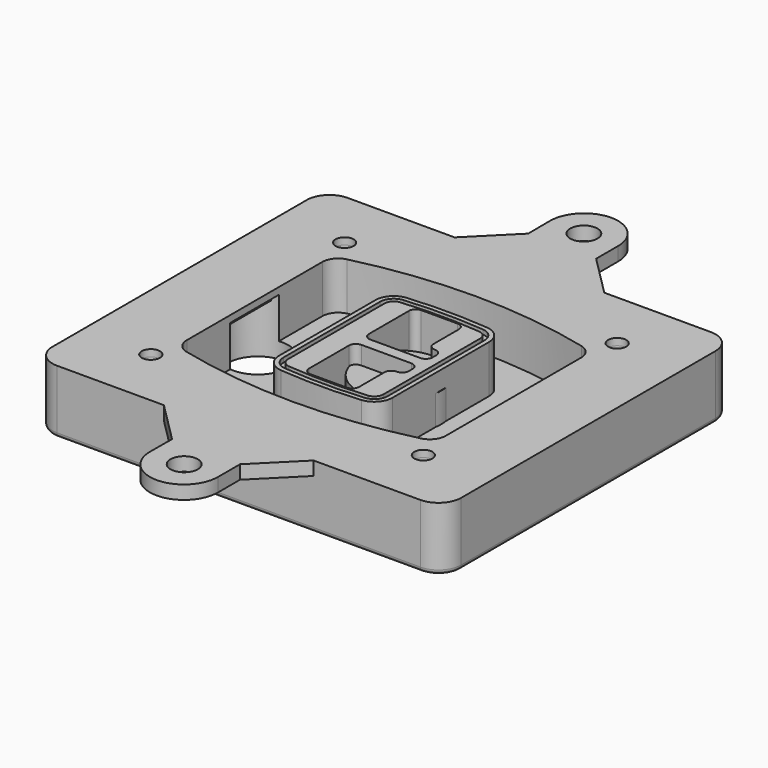
from build123d import *

# Parameters (mm, degrees)
F0_R      = 4
F1_DEPTH  = 25
F2_DEPTH  = 3
F3_DEPTH  = 18
F5_DEPTH  = 21
F6_DEPTH  = 2
F8_DEPTH  = 20
F9_DEPTH  = 16
F10_DEPTH = 25
F7_R      = 6
F7_R_2    = 4
F11_DEPTH = 6
F13_DEPTH = 9
F15_R     = 2
F16_R     = 4
F16_R_2   = 6
F17_DEPTH = 3


# Not quite as in the source:
# - a feature of the source that left no trace in its solid (it failed there, or was rolled back) is left out
# - a feature names something its author has since deleted; it is built from what else it names


with BuildPart() as f1:
    # F0 (on Top) → F1 (new body)
    with BuildSketch(Plane.XY):
        with BuildLine():
            ThreePointArc((-90, -70), (-87.0710678119, -77.0710678119), (-80, -80))
            Line((-80, -80), (80, -80))
            ThreePointArc((80, -80), (87.0710678119, -77.0710678119), (90, -70))
            Line((90, -70), (90, 70))
            ThreePointArc((90, 70), (87.0710678119, 77.0710678119), (80, 80))
            Line((80, 80), (-80, 80))
            ThreePointArc((-80, 80), (-87.0710678119, 77.0710678119), (-90, 70))
            Line((-90, 70), (-90, -70))
        make_face()
        with Locations((-60, -53.3333333333)):
            Circle(F0_R, mode=Mode.SUBTRACT)
        with Locations((60, -53.3333333333)):
            Circle(F0_R, mode=Mode.SUBTRACT)
        with BuildLine():
            ThreePointArc((-64, 37.2990447398), (-61.0143011354, 45.9411029726), (-53.3306899286, 50.8970778549))
            ThreePointArc((-53.3306899286, 50.8970778549), (0, 57.3333333333), (53.3306899286, 50.8970778549))
            ThreePointArc((53.3306899286, 50.8970778549), (61.0143011354, 45.9411029726), (64, 37.2990447398))
            Line((64, 37.2990447398), (64, -37.2990447398))
            ThreePointArc((64, -37.2990447398), (61.0143011354, -45.9411029726), (53.3306899286, -50.8970778549))
            ThreePointArc((53.3306899286, -50.8970778549), (0, -57.3333333333), (-53.3306899286, -50.8970778549))
            ThreePointArc((-53.3306899286, -50.8970778549), (-61.0143011354, -45.9411029726), (-64, -37.2990447398))
            Line((-64, -37.2990447398), (-64, 37.2990447398))
        make_face(mode=Mode.SUBTRACT)
        with Locations((-60, 53.3333333333)):
            Circle(F0_R, mode=Mode.SUBTRACT)
        with Locations((60, 53.3333333333)):
            Circle(F0_R, mode=Mode.SUBTRACT)
        with BuildLine():
            ThreePointArc((53.3306899286, 50.8970778549), (0, 57.3333333333), (-53.3306899286, 50.8970778549))
            ThreePointArc((-53.3306899286, 50.8970778549), (-61.0143011354, 45.9411029726), (-64, 37.2990447398))
            Line((-64, 37.2990447398), (-64, -37.2990447398))
            ThreePointArc((-64, -37.2990447398), (-61.0143011354, -45.9411029726), (-53.3306899286, -50.8970778549))
            ThreePointArc((-53.3306899286, -50.8970778549), (0, -57.3333333333), (53.3306899286, -50.8970778549))
            ThreePointArc((53.3306899286, -50.8970778549), (61.0143011354, -45.9411029726), (64, -37.2990447398))
            Line((64, -37.2990447398), (64, 37.2990447398))
            ThreePointArc((64, 37.2990447398), (61.0143011354, 45.9411029726), (53.3306899286, 50.8970778549))
        make_face()
        with BuildLine():
            Line((-60, -37.2990447398), (-60, 37.2990447398))
            ThreePointArc((-60, 37.2990447398), (-57.8673579538, 43.4719434775), (-52.3790642347, 47.0119255363))
            ThreePointArc((-52.3790642347, 47.0119255363), (0, 53.3333333333), (52.3790642347, 47.0119255363))
            ThreePointArc((52.3790642347, 47.0119255363), (57.8673579538, 43.4719434775), (60, 37.2990447398))
            Line((60, 37.2990447398), (60, -37.2990447398))
            ThreePointArc((60, -37.2990447398), (57.8673579538, -43.4719434775), (52.3790642347, -47.0119255363))
            ThreePointArc((52.3790642347, -47.0119255363), (0, -53.3333333333), (-52.3790642347, -47.0119255363))
            ThreePointArc((-52.3790642347, -47.0119255363), (-57.8673579538, -43.4719434775), (-60, -37.2990447398))
        make_face(mode=Mode.SUBTRACT)
        with BuildLine():
            ThreePointArc((-52.3790642347, 47.0119255363), (-57.8673579538, 43.4719434775), (-60, 37.2990447398))
            Line((-60, 37.2990447398), (-60, -37.2990447398))
            ThreePointArc((-60, -37.2990447398), (-57.8673579538, -43.4719434775), (-52.3790642347, -47.0119255363))
            ThreePointArc((-52.3790642347, -47.0119255363), (0, -53.3333333333), (52.3790642347, -47.0119255363))
            ThreePointArc((52.3790642347, -47.0119255363), (57.8673579538, -43.4719434775), (60, -37.2990447398))
            Line((60, -37.2990447398), (60, 37.2990447398))
            ThreePointArc((60, 37.2990447398), (57.8673579538, 43.4719434775), (52.3790642347, 47.0119255363))
            ThreePointArc((52.3790642347, 47.0119255363), (0, 53.3333333333), (-52.3790642347, 47.0119255363))
        make_face()
        with BuildLine():
            ThreePointArc((51.6653449643, 44.0980612973), (55.5071505677, 41.6200738562), (57, 37.2990447398))
            Line((57, 37.2990447398), (57, -37.2990447398))
            ThreePointArc((57, -37.2990447398), (55.5071505677, -41.6200738562), (51.6653449643, -44.0980612973))
            ThreePointArc((51.6653449643, -44.0980612973), (0, -50.3333333333), (-51.6653449643, -44.0980612973))
            ThreePointArc((-51.6653449643, -44.0980612973), (-55.5071505677, -41.6200738562), (-57, -37.2990447398))
            Line((-57, -37.2990447398), (-57, 37.2990447398))
            ThreePointArc((-57, 37.2990447398), (-55.5071505677, 41.6200738562), (-51.6653449643, 44.0980612973))
            ThreePointArc((-51.6653449643, 44.0980612973), (0, 50.3333333333), (51.6653449643, 44.0980612973))
        make_face(mode=Mode.SUBTRACT)
        with BuildLine():
            Line((57, -37.2990447398), (57, 37.2990447398))
            ThreePointArc((57, 37.2990447398), (55.5071505677, 41.6200738562), (51.6653449643, 44.0980612973))
            ThreePointArc((51.6653449643, 44.0980612973), (0, 50.3333333333), (-51.6653449643, 44.0980612973))
            ThreePointArc((-51.6653449643, 44.0980612973), (-55.5071505677, 41.6200738562), (-57, 37.2990447398))
            Line((-57, 37.2990447398), (-57, -37.2990447398))
            ThreePointArc((-57, -37.2990447398), (-55.5071505677, -41.6200738562), (-51.6653449643, -44.0980612973))
            ThreePointArc((-51.6653449643, -44.0980612973), (0, -50.3333333333), (51.6653449643, -44.0980612973))
            ThreePointArc((51.6653449643, -44.0980612973), (55.5071505677, -41.6200738562), (57, -37.2990447398))
        make_face()
    extrude(amount=-F1_DEPTH)

    # F0 (on Top) → F2 (join)
    with BuildSketch(Plane.XY):
        with BuildLine():
            ThreePointArc((-52.3790642347, 47.0119255363), (-57.8673579538, 43.4719434775), (-60, 37.2990447398))
            Line((-60, 37.2990447398), (-60, -37.2990447398))
            ThreePointArc((-60, -37.2990447398), (-57.8673579538, -43.4719434775), (-52.3790642347, -47.0119255363))
            ThreePointArc((-52.3790642347, -47.0119255363), (0, -53.3333333333), (52.3790642347, -47.0119255363))
            ThreePointArc((52.3790642347, -47.0119255363), (57.8673579538, -43.4719434775), (60, -37.2990447398))
            Line((60, -37.2990447398), (60, 37.2990447398))
            ThreePointArc((60, 37.2990447398), (57.8673579538, 43.4719434775), (52.3790642347, 47.0119255363))
            ThreePointArc((52.3790642347, 47.0119255363), (0, 53.3333333333), (-52.3790642347, 47.0119255363))
        make_face()
        with BuildLine():
            ThreePointArc((51.6653449643, 44.0980612973), (55.5071505677, 41.6200738562), (57, 37.2990447398))
            Line((57, 37.2990447398), (57, -37.2990447398))
            ThreePointArc((57, -37.2990447398), (55.5071505677, -41.6200738562), (51.6653449643, -44.0980612973))
            ThreePointArc((51.6653449643, -44.0980612973), (0, -50.3333333333), (-51.6653449643, -44.0980612973))
            ThreePointArc((-51.6653449643, -44.0980612973), (-55.5071505677, -41.6200738562), (-57, -37.2990447398))
            Line((-57, -37.2990447398), (-57, 37.2990447398))
            ThreePointArc((-57, 37.2990447398), (-55.5071505677, 41.6200738562), (-51.6653449643, 44.0980612973))
            ThreePointArc((-51.6653449643, 44.0980612973), (0, 50.3333333333), (51.6653449643, 44.0980612973))
        make_face(mode=Mode.SUBTRACT)
    extrude(amount=F2_DEPTH)

    # F0 (on Top) → F3 (cut)
    with BuildSketch(Plane.XY):
        with BuildLine():
            Line((57, -37.2990447398), (57, 37.2990447398))
            ThreePointArc((57, 37.2990447398), (55.5071505677, 41.6200738562), (51.6653449643, 44.0980612973))
            ThreePointArc((51.6653449643, 44.0980612973), (0, 50.3333333333), (-51.6653449643, 44.0980612973))
            ThreePointArc((-51.6653449643, 44.0980612973), (-55.5071505677, 41.6200738562), (-57, 37.2990447398))
            Line((-57, 37.2990447398), (-57, -37.2990447398))
            ThreePointArc((-57, -37.2990447398), (-55.5071505677, -41.6200738562), (-51.6653449643, -44.0980612973))
            ThreePointArc((-51.6653449643, -44.0980612973), (0, -50.3333333333), (51.6653449643, -44.0980612973))
            ThreePointArc((51.6653449643, -44.0980612973), (55.5071505677, -41.6200738562), (57, -37.2990447398))
        make_face()
    extrude(amount=-F3_DEPTH, mode=Mode.SUBTRACT)

    # F4 (on face) → F5 (join, through all)
    with BuildSketch(Plane.XY.offset(3)):
        with BuildLine():
            ThreePointArc((-25, -26.587695628), (-22.8992979869, -31.9912392117), (-17.7004291845, -34.5569740744))
            ThreePointArc((-17.7004291845, -34.5569740744), (0, -35.3333333333), (17.7004291845, -34.5569740744))
            ThreePointArc((17.7004291845, -34.5569740744), (22.8992979869, -31.9912392117), (25, -26.587695628))
            Line((25, -26.587695628), (25, 26.587695628))
            ThreePointArc((25, 26.587695628), (22.8992979869, 31.9912392117), (17.7004291845, 34.5569740744))
            ThreePointArc((17.7004291845, 34.5569740744), (0, 35.3333333333), (-17.7004291845, 34.5569740744))
            ThreePointArc((-17.7004291845, 34.5569740744), (-22.8992979869, 31.9912392117), (-25, 26.587695628))
            Line((-25, 26.587695628), (-25, -26.587695628))
        make_face()
        with BuildLine():
            ThreePointArc((17.5253218884, 32.5646544628), (21.4244734902, 30.6403533158), (23, 26.587695628))
            Line((23, 26.587695628), (23, -26.587695628))
            ThreePointArc((23, -26.587695628), (21.4244734902, -30.6403533158), (17.5253218884, -32.5646544628))
            ThreePointArc((17.5253218884, -32.5646544628), (0, -33.3333333333), (-17.5253218884, -32.5646544628))
            ThreePointArc((-17.5253218884, -32.5646544628), (-21.4244734902, -30.6403533158), (-23, -26.587695628))
            Line((-23, -26.587695628), (-23, 26.587695628))
            ThreePointArc((-23, 26.587695628), (-21.4244734902, 30.6403533158), (-17.5253218884, 32.5646544628))
            ThreePointArc((-17.5253218884, 32.5646544628), (0, 33.3333333333), (17.5253218884, 32.5646544628))
        make_face(mode=Mode.SUBTRACT)
        with BuildLine():
            Line((23, -26.587695628), (23, 26.587695628))
            ThreePointArc((23, 26.587695628), (21.4244734902, 30.6403533158), (17.5253218884, 32.5646544628))
            ThreePointArc((17.5253218884, 32.5646544628), (0, 33.3333333333), (-17.5253218884, 32.5646544628))
            ThreePointArc((-17.5253218884, 32.5646544628), (-21.4244734902, 30.6403533158), (-23, 26.587695628))
            Line((-23, 26.587695628), (-23, -26.587695628))
            ThreePointArc((-23, -26.587695628), (-21.4244734902, -30.6403533158), (-17.5253218884, -32.5646544628))
            ThreePointArc((-17.5253218884, -32.5646544628), (0, -33.3333333333), (17.5253218884, -32.5646544628))
            ThreePointArc((17.5253218884, -32.5646544628), (21.4244734902, -30.6403533158), (23, -26.587695628))
        make_face()
        with BuildLine():
            ThreePointArc((17.3502145923, 30.5723348512), (19.9496489934, 29.2894674198), (21, 26.587695628))
            Line((21, 26.587695628), (21, -26.587695628))
            ThreePointArc((21, -26.587695628), (19.9496489934, -29.2894674198), (17.3502145923, -30.5723348512))
            ThreePointArc((17.3502145923, -30.5723348512), (0, -31.3333333333), (-17.3502145923, -30.5723348512))
            ThreePointArc((-17.3502145923, -30.5723348512), (-19.9496489934, -29.2894674198), (-21, -26.587695628))
            Line((-21, -26.587695628), (-21, 26.587695628))
            ThreePointArc((-21, 26.587695628), (-19.9496489934, 29.2894674198), (-17.3502145923, 30.5723348512))
            ThreePointArc((-17.3502145923, 30.5723348512), (0, 31.3333333333), (17.3502145923, 30.5723348512))
        make_face(mode=Mode.SUBTRACT)
        with BuildLine():
            Line((21, -26.587695628), (21, 26.587695628))
            ThreePointArc((21, 26.587695628), (19.9496489934, 29.2894674198), (17.3502145923, 30.5723348512))
            ThreePointArc((17.3502145923, 30.5723348512), (0, 31.3333333333), (-17.3502145923, 30.5723348512))
            ThreePointArc((-17.3502145923, 30.5723348512), (-19.9496489934, 29.2894674198), (-21, 26.587695628))
            Line((-21, 26.587695628), (-21, -26.587695628))
            ThreePointArc((-21, -26.587695628), (-19.9496489934, -29.2894674198), (-17.3502145923, -30.5723348512))
            ThreePointArc((-17.3502145923, -30.5723348512), (0, -31.3333333333), (17.3502145923, -30.5723348512))
            ThreePointArc((17.3502145923, -30.5723348512), (19.9496489934, -29.2894674198), (21, -26.587695628))
        make_face()
        with BuildLine():
            Line((-8, -2.5), (14, -2.5))
            ThreePointArc((14, -2.5), (16.1213203436, -3.3786796564), (17, -5.5))
            Line((17, -5.5), (17, -7.5))
            ThreePointArc((17, -7.5), (16.1213203436, -9.6213203436), (14, -10.5))
            ThreePointArc((14, -10.5), (11.8786796564, -11.3786796564), (11, -13.5))
            Line((11, -13.5), (11, -27.5))
            ThreePointArc((11, -27.5), (10.1213203436, -29.6213203436), (8, -30.5))
            Line((8, -30.5), (-8, -30.5))
            ThreePointArc((-8, -30.5), (-10.1213203436, -29.6213203436), (-11, -27.5))
            Line((-11, -27.5), (-11, -5.5))
            ThreePointArc((-11, -5.5), (-10.1213203436, -3.3786796564), (-8, -2.5))
        make_face(mode=Mode.SUBTRACT)
        with BuildLine():
            ThreePointArc((-8, 2.5), (-10.1213203436, 3.3786796564), (-11, 5.5))
            Line((-11, 5.5), (-11, 27.5))
            ThreePointArc((-11, 27.5), (-10.1213203436, 29.6213203436), (-8, 30.5))
            Line((-8, 30.5), (8, 30.5))
            ThreePointArc((8, 30.5), (10.1213203436, 29.6213203436), (11, 27.5))
            Line((11, 27.5), (11, 13.5))
            ThreePointArc((11, 13.5), (11.8786796564, 11.3786796564), (14, 10.5))
            ThreePointArc((14, 10.5), (16.1213203436, 9.6213203436), (17, 7.5))
            Line((17, 7.5), (17, 5.5))
            ThreePointArc((17, 5.5), (16.1213203436, 3.3786796564), (14, 2.5))
            Line((14, 2.5), (-8, 2.5))
        make_face(mode=Mode.SUBTRACT)
    extrude(amount=-F5_DEPTH)

    # F4 (on face) → F6 (cut)
    with BuildSketch(Plane.XY.offset(3)):
        with BuildLine():
            Line((23, -26.587695628), (23, 26.587695628))
            ThreePointArc((23, 26.587695628), (21.4244734902, 30.6403533158), (17.5253218884, 32.5646544628))
            ThreePointArc((17.5253218884, 32.5646544628), (0, 33.3333333333), (-17.5253218884, 32.5646544628))
            ThreePointArc((-17.5253218884, 32.5646544628), (-21.4244734902, 30.6403533158), (-23, 26.587695628))
            Line((-23, 26.587695628), (-23, -26.587695628))
            ThreePointArc((-23, -26.587695628), (-21.4244734902, -30.6403533158), (-17.5253218884, -32.5646544628))
            ThreePointArc((-17.5253218884, -32.5646544628), (0, -33.3333333333), (17.5253218884, -32.5646544628))
            ThreePointArc((17.5253218884, -32.5646544628), (21.4244734902, -30.6403533158), (23, -26.587695628))
        make_face()
        with BuildLine():
            ThreePointArc((17.3502145923, 30.5723348512), (19.9496489934, 29.2894674198), (21, 26.587695628))
            Line((21, 26.587695628), (21, -26.587695628))
            ThreePointArc((21, -26.587695628), (19.9496489934, -29.2894674198), (17.3502145923, -30.5723348512))
            ThreePointArc((17.3502145923, -30.5723348512), (0, -31.3333333333), (-17.3502145923, -30.5723348512))
            ThreePointArc((-17.3502145923, -30.5723348512), (-19.9496489934, -29.2894674198), (-21, -26.587695628))
            Line((-21, -26.587695628), (-21, 26.587695628))
            ThreePointArc((-21, 26.587695628), (-19.9496489934, 29.2894674198), (-17.3502145923, 30.5723348512))
            ThreePointArc((-17.3502145923, 30.5723348512), (0, 31.3333333333), (17.3502145923, 30.5723348512))
        make_face(mode=Mode.SUBTRACT)
    extrude(amount=-F6_DEPTH, mode=Mode.SUBTRACT)

    # F7 (on face) → F8 (join)
    with BuildSketch(Plane(origin=(0, 0, -25), x_dir=(1, 0, 0), z_dir=(0, 0, -1))):
        with BuildLine():
            ThreePointArc((-6.71157564, 0), (6.7567035675, 13.4682792075), (20.224982775, 0))
            Line((20.224982775, 0), (25.224982775, 0))
            ThreePointArc((25.224982775, 0), (6.7567035675, 18.4682792075), (-11.71157564, 0))
            Line((-11.71157564, 0), (-6.71157564, 0))
        make_face()
        with BuildLine():
            Line((-6.71157564, 0), (20.224982775, 0))
            ThreePointArc((20.224982775, 0), (6.7567035675, 13.4682792075), (-6.71157564, 0))
        make_face()
        with BuildLine():
            ThreePointArc((-6.71157564, 0), (6.7567035675, -13.4682792075), (20.224982775, 0))
            Line((20.224982775, 0), (-6.71157564, 0))
        make_face()
        with BuildLine():
            Line((25.224982775, 0), (20.224982775, 0))
            ThreePointArc((20.224982775, 0), (6.7567035675, -13.4682792075), (-6.71157564, 0))
            Line((-6.71157564, 0), (-11.71157564, 0))
            ThreePointArc((-11.71157564, 0), (6.7567035675, -18.4682792075), (25.224982775, 0))
        make_face()
    extrude(amount=-F8_DEPTH)

    # F7 (on face) → F9 (cut)
    with BuildSketch(Plane(origin=(0, 0, -25), x_dir=(1, 0, 0), z_dir=(0, 0, -1))):
        with BuildLine():
            Line((-6.71157564, 0), (20.224982775, 0))
            ThreePointArc((20.224982775, 0), (6.7567035675, 13.4682792075), (-6.71157564, 0))
        make_face()
        with BuildLine():
            ThreePointArc((-6.71157564, 0), (6.7567035675, -13.4682792075), (20.224982775, 0))
            Line((20.224982775, 0), (-6.71157564, 0))
        make_face()
    extrude(amount=-F9_DEPTH, mode=Mode.SUBTRACT)

    # F7 (on face) → F10 (cut)
    with BuildSketch(Plane(origin=(0, 0, -25), x_dir=(1, 0, 0), z_dir=(0, 0, -1))):
        with BuildLine():
            Line((-69.0318229325, 0), (-42.0952645175, 0))
            ThreePointArc((-42.0952645175, 0), (-55.563543725, 13.4682792075), (-69.0318229325, 0))
        make_face()
        with BuildLine():
            ThreePointArc((-69.0318229325, 0), (-55.563543725, -13.4682792075), (-42.0952645175, 0))
            Line((-42.0952645175, 0), (-69.0318229325, 0))
        make_face()
    extrude(amount=-F10_DEPTH, mode=Mode.SUBTRACT)

    # F7 (on face) → F11 (cut)
    with BuildSketch(Plane(origin=(0, 0, -25), x_dir=(1, 0, 0), z_dir=(0, 0, -1))):
        with Locations((60, -53.3333333333)):
            Circle(F7_R)
        with Locations((60, -53.3333333333)):
            Circle(F7_R_2, mode=Mode.SUBTRACT)
        with Locations((-60, -53.3333333333)):
            Circle(F7_R)
        with Locations((-60, -53.3333333333)):
            Circle(F7_R_2, mode=Mode.SUBTRACT)
        with Locations((-60, 53.3333333333)):
            Circle(F7_R)
        with Locations((-60, 53.3333333333)):
            Circle(F7_R_2, mode=Mode.SUBTRACT)
        with Locations((60, 53.3333333333)):
            Circle(F7_R)
        with Locations((60, 53.3333333333)):
            Circle(F7_R_2, mode=Mode.SUBTRACT)
    extrude(amount=-F11_DEPTH, mode=Mode.SUBTRACT)

    # F12 (on face) → F13 (cut, through all)
    with BuildSketch(Plane(origin=(0, 0, -9), x_dir=(1, 0, 0), z_dir=(0, 0, -1))):
        with BuildLine():
            ThreePointArc((20.224982775, 0), (20.1663399806, 1.2554664788), (19.9909222755, 2.5))
            Line((19.9909222755, 2.5), (14, 2.5))
            ThreePointArc((14, 2.5), (16.1213203436, 3.3786796564), (17, 5.5))
            Line((17, 5.5), (17, 7.5))
            ThreePointArc((17, 7.5), (16.1213203436, 9.6213203436), (14, 10.5))
            ThreePointArc((14, 10.5), (12.1627255951, 11.1284134507), (11.0951631559, 12.750384826))
            ThreePointArc((11.0951631559, 12.750384826), (11.0476113807, 12.7664660322), (11, 12.7823698976))
            Line((11, 12.7823698976), (11, -12.7823698976))
            ThreePointArc((11, -12.7823698976), (11.0476113807, -12.7664660322), (11.0951631559, -12.750384826))
            ThreePointArc((11.0951631559, -12.750384826), (12.1627255951, -11.1284134507), (14, -10.5))
            ThreePointArc((14, -10.5), (16.1213203436, -9.6213203436), (17, -7.5))
            Line((17, -7.5), (17, -5.5))
            ThreePointArc((17, -5.5), (16.1213203436, -3.3786796564), (14, -2.5))
            Line((14, -2.5), (19.9909222755, -2.5))
            ThreePointArc((19.9909222755, -2.5), (20.1663399806, -1.2554664788), (20.224982775, 0))
        make_face()
    extrude(amount=F13_DEPTH, mode=Mode.SUBTRACT)

    # F15
    f15_edges = [f1.edges().sort_by_distance(p)[0] for p in [
        (0, -80, -25),
        (-87.071068, -77.071068, -25),
        (-90, 0, -25),
        (-87.071068, 77.071068, -25),
        (87.071068, -77.071068, -25),
        (0, 80, -25),
        (90, 0, -25),
        (87.071068, 77.071068, -25),
    ]]
    fillet(f15_edges, radius=F15_R)

    # F16 (on Top) → F17 (join, symmetric)
    with BuildSketch(Plane.XY):
        with BuildLine():
            Line((-32.9200348033, 80), (-80, 80))
            ThreePointArc((-80, 80), (-87.0710678119, 77.0710678119), (-90, 70))
            Line((-90, 70), (-90, -70))
            ThreePointArc((-90, -70), (-87.0710678119, -77.0710678119), (-80, -80))
            Line((-80, -80), (-32.9200348033, -80))
            Line((-32.9200348033, -80), (32.9998691691, -80))
            Line((32.9998691691, -80), (80, -80))
            ThreePointArc((80, -80), (87.0710678119, -77.0710678119), (90, -70))
            Line((90, -70), (90, 70))
            ThreePointArc((90, 70), (87.0710678119, 77.0710678119), (80, 80))
            Line((80, 80), (32.9998691691, 80))
            Line((32.9998691691, 80), (-32.9200348033, 80))
        make_face()
        with Locations((-60, -53.3333333333)):
            Circle(F16_R, mode=Mode.SUBTRACT)
        with Locations((60, -53.3333333333)):
            Circle(F16_R, mode=Mode.SUBTRACT)
        with Locations((-60, 53.3333333333)):
            Circle(F16_R, mode=Mode.SUBTRACT)
        with BuildLine():
            ThreePointArc((-52.3790642347, 47.0119255363), (0, 53.3333333333), (52.3790642347, 47.0119255363))
            ThreePointArc((52.3790642347, 47.0119255363), (57.8673579538, 43.4719434775), (60, 37.2990447398))
            Line((60, 37.2990447398), (60, -37.2990447398))
            ThreePointArc((60, -37.2990447398), (57.8673579538, -43.4719434775), (52.3790642347, -47.0119255363))
            ThreePointArc((52.3790642347, -47.0119255363), (0, -53.3333333333), (-52.3790642347, -47.0119255363))
            ThreePointArc((-52.3790642347, -47.0119255363), (-57.8673579538, -43.4719434775), (-60, -37.2990447398))
            Line((-60, -37.2990447398), (-60, 37.2990447398))
            ThreePointArc((-60, 37.2990447398), (-57.8673579538, 43.4719434775), (-52.3790642347, 47.0119255363))
        make_face(mode=Mode.SUBTRACT)
        with Locations((60, 53.3333333333)):
            Circle(F16_R, mode=Mode.SUBTRACT)
        with BuildLine():
            Line((-14.9200993547, 98), (-32.9200348033, 80))
            Line((-32.9200348033, 80), (32.9998691691, 80))
            Line((32.9998691691, 80), (15.0000000006, 97.9998691685))
            Line((15.0000000006, 97.9998691685), (15.0000000006, 109.9998691685))
            ThreePointArc((15.0000000006, 109.9998691685), (0.0003270806, 125.0989261942), (-14.9993458393, 109.9998691685))
            Line((-14.9993458393, 109.9998691685), (-14.9200993547, 98))
        make_face()
        with Locations((0, 110)):
            Circle(F16_R_2, mode=Mode.SUBTRACT)
        with BuildLine():
            Line((32.9998691691, -80), (-32.9200348033, -80))
            Line((-32.9200348033, -80), (-14.9200993547, -98))
            Line((-14.9200993547, -98), (-14.9993458393, -109.9998691685))
            ThreePointArc((-14.9993458393, -109.9998691685), (0.0003270806, -125.0989261942), (15.0000000006, -109.9998691685))
            Line((15.0000000006, -109.9998691685), (15.0000000006, -97.9998691685))
            Line((15.0000000006, -97.9998691685), (32.9998691691, -80))
        make_face()
        with Locations((0, -110)):
            Circle(F16_R_2, mode=Mode.SUBTRACT)
    extrude(amount=F17_DEPTH, both=True)


solid = f1.part
